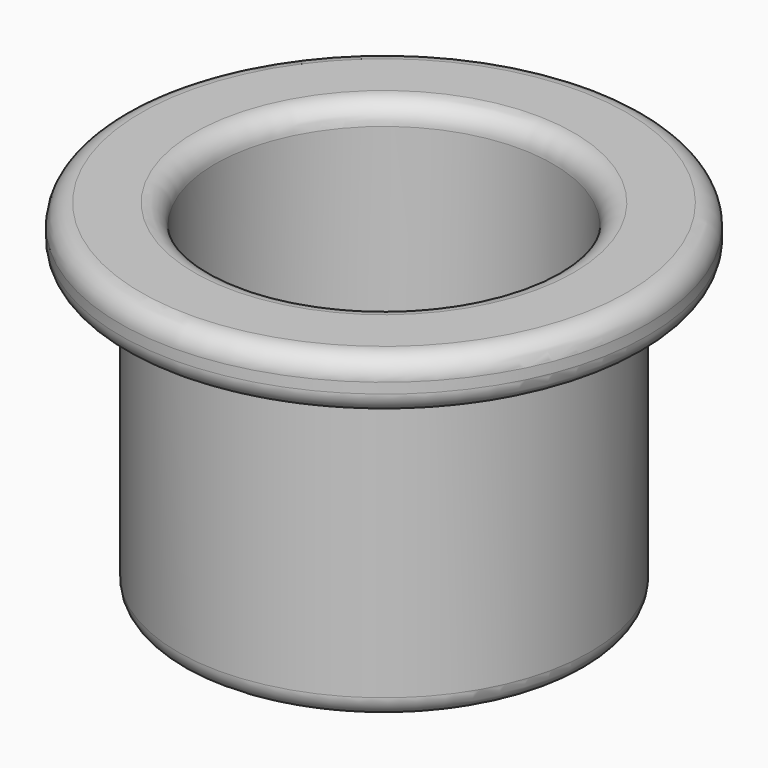
from build123d import *

# Parameters (mm, degrees)
F0_R     = 7.9375
F0_R_2   = 6.5
F1_DEPTH = 11.43
F2_R     = 10.16
F2_R_2   = 6.5
F3_DEPTH = 2
F4_R     = 0.8


# Not quite as in the source:
# - a fillet or chamfer that OpenCascade refuses, or shapes differently, is made with other operations: its cross-section is extruded or revolved along the edge and cut away or added


with BuildPart() as f1:
    # F0 (on Top) → F1 (new body)
    with BuildSketch(Plane.XY):
        Circle(F0_R)
        Circle(F0_R_2, mode=Mode.SUBTRACT)
    extrude(amount=F1_DEPTH)

    # F2 (on face) → F3 (join)
    with BuildSketch(Plane.XY.offset(11.43)):
        Circle(F2_R)
        Circle(F2_R_2, mode=Mode.SUBTRACT)
    extrude(amount=F3_DEPTH)

    # F4
    f4_edges = [f1.edges().sort_by_distance(p)[0] for p in [
        (-6.5, 0, 13.43),
        (-6.5, 0, 0),
        (-7.9375, 0, 11.43),
        (-10.16, 0, 13.43),
    ]]
    fillet(f4_edges, radius=F4_R)

    # F5: fillet of radius 0.8 on 2 edges, made by hand

    # F5_s1 → F5_t2 (revolve, cut)
    with BuildSketch(Plane.XZ):
        with BuildLine():
            ThreePointArc((7.9375, 0.7833222517), (7.7579836823, 0.2783470048), (7.3, 0))
            Line((7.3, 0), (7.9375, 0))
            Line((7.9375, 0), (7.9375, 0.7833222517))
        make_face()
    revolve(axis=Axis((0, 0, 0), (0, 0, 1)), mode=Mode.SUBTRACT)

    # F5_s3 → F5_t4 (revolve, cut)
    with BuildSketch(Plane.XZ):
        with BuildLine():
            ThreePointArc((9.36, 11.43), (9.9256854249, 11.6643145751), (10.16, 12.23))
            Line((10.16, 12.23), (10.16, 11.43))
            Line((10.16, 11.43), (9.36, 11.43))
        make_face()
    revolve(axis=Axis((0, 0, 11.43), (0, 0, 1)), mode=Mode.SUBTRACT)


solid = f1.part
